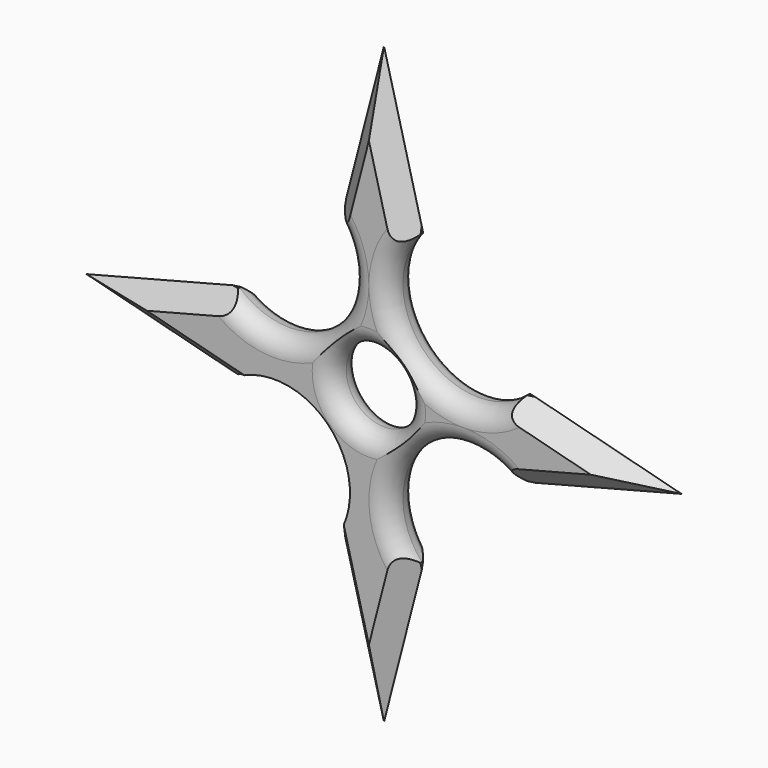
from build123d import *

# Parameters (mm, degrees)
F0_W         = 19.05
F0_H         = 25.4
F0_W_2       = 25.4
F0_H_2       = 19.05
F1_DEPTH     = 12.7
F3_D         = 50.8
F4_SIZE2     = 6.34999
F4_SIZE      = 6.34999
F5_T6_ANGLE  = 208.6059171241
F5_T8_ANGLE  = 208.6059171241
F5_T10_ANGLE = 208.6059171241
F5_T12_ANGLE = 208.6059171241
F5_T14_ANGLE = 208.6059171241
F5_T16_ANGLE = 208.6059171241
F5_T18_ANGLE = 208.6059171241


# Not quite as in the source:
# - a fillet or chamfer that OpenCascade refuses, or shapes differently, is made with other operations: its cross-section is extruded or revolved along the edge and cut away or added
# - a fillet or chamfer is up to 0.001 mm smaller than in the source, because OpenCascade refuses the exact size


with BuildPart() as f1:
    # F0 (on Front) → F1 (new body)
    with BuildSketch(Plane.XZ):
        with BuildLine():
            Line((-12.7, 12.7), (-4.87e-08, 12.7))
            Line((-4.87e-08, 12.7), (12.7, 12.7))
            Line((12.7, 12.7), (12.7, 14.1990316571))
            ThreePointArc((12.7, 14.1990316571), (0, 19.05), (-12.7, 14.1990316571))
            Line((-12.7, 14.1990316571), (-12.7, 12.7))
        make_face()
        with BuildLine():
            Line((-12.7, -12.7), (-12.7, 0))
            Line((-12.7, 0), (-12.7, 12.7))
            Line((-12.7, 12.7), (-14.1990316571, 12.7))
            ThreePointArc((-14.1990316571, 12.7), (-19.05, 0), (-14.1990316571, -12.7))
            Line((-14.1990316571, -12.7), (-12.7, -12.7))
        make_face()
        with BuildLine():
            Line((12.7, -12.7), (6e-10, -12.7))
            Line((6e-10, -12.7), (-12.7, -12.7))
            Line((-12.7, -12.7), (-12.7, -14.1990316571))
            ThreePointArc((-12.7, -14.1990316571), (0, -19.05), (12.7, -14.1990316571))
            Line((12.7, -14.1990316571), (12.7, -12.7))
        make_face()
        with BuildLine():
            Line((12.7, 12.7), (12.7, 0))
            Line((12.7, 0), (12.7, -12.7))
            Line((12.7, -12.7), (14.1990316571, -12.7))
            ThreePointArc((14.1990316571, -12.7), (17.7959834382, -6.7974608102), (19.05, 0))
            ThreePointArc((19.05, 0), (17.7959834382, 6.7974608102), (14.1990316571, 12.7))
            Line((14.1990316571, 12.7), (12.7, 12.7))
        make_face()
        with BuildLine():
            Line((12.7, -12.7), (12.7, 0))
            ThreePointArc((12.7, 0), (8.9802561213, -8.9802561208), (6e-10, -12.7))
            Line((6e-10, -12.7), (12.7, -12.7))
        make_face()
        with BuildLine():
            Line((-12.7, -12.7), (6e-10, -12.7))
            ThreePointArc((6e-10, -12.7), (-8.9802561208, -8.9802561213), (-12.7, 0))
            Line((-12.7, 0), (-12.7, -12.7))
        make_face()
        with BuildLine():
            ThreePointArc((-12.7, 0), (-8.9802561383, 8.9802561039), (-4.87e-08, 12.7))
            Line((-4.87e-08, 12.7), (-12.7, 12.7))
            Line((-12.7, 12.7), (-12.7, 0))
        make_face()
        with BuildLine():
            ThreePointArc((-4.87e-08, 12.7), (8.9802561039, 8.9802561383), (12.7, 0))
            Line((12.7, 0), (12.7, 12.7))
            Line((12.7, 12.7), (-4.87e-08, 12.7))
        make_face()
        with BuildLine():
            Line((12.7, 31.75), (12.7, 14.1990316571))
            ThreePointArc((12.7, 14.1990316571), (13.4703841816, 13.4703841816), (14.1990316571, 12.7))
            Line((14.1990316571, 12.7), (31.75, 12.7))
            Line((31.75, 12.7), (31.75, 31.75))
            Line((31.75, 31.75), (12.7, 31.75))
        make_face()
        with BuildLine():
            ThreePointArc((-12.7, 14.1990316571), (0, 19.05), (12.7, 14.1990316571))
            Line((12.7, 14.1990316571), (12.7, 31.75))
            Line((12.7, 31.75), (-12.7, 31.75))
            Line((-12.7, 31.75), (-12.7, 14.1990316571))
        make_face()
        with BuildLine():
            ThreePointArc((-14.1990316571, 12.7), (-13.4703841816, 13.4703841816), (-12.7, 14.1990316571))
            Line((-12.7, 14.1990316571), (-12.7, 31.75))
            Line((-12.7, 31.75), (-31.75, 31.75))
            Line((-31.75, 31.75), (-31.75, 12.7))
            Line((-31.75, 12.7), (-14.1990316571, 12.7))
        make_face()
        with BuildLine():
            ThreePointArc((-14.1990316571, -12.7), (-19.05, 0), (-14.1990316571, 12.7))
            Line((-14.1990316571, 12.7), (-31.75, 12.7))
            Line((-31.75, 12.7), (-31.75, -12.7))
            Line((-31.75, -12.7), (-14.1990316571, -12.7))
        make_face()
        with BuildLine():
            Line((-12.7, -31.75), (-12.7, -14.1990316571))
            ThreePointArc((-12.7, -14.1990316571), (-13.4703841816, -13.4703841816), (-14.1990316571, -12.7))
            Line((-14.1990316571, -12.7), (-31.75, -12.7))
            Line((-31.75, -12.7), (-31.75, -31.75))
            Line((-31.75, -31.75), (-12.7, -31.75))
        make_face()
        with BuildLine():
            Line((12.7, -31.75), (12.7, -14.1990316571))
            ThreePointArc((12.7, -14.1990316571), (0, -19.05), (-12.7, -14.1990316571))
            Line((-12.7, -14.1990316571), (-12.7, -31.75))
            Line((-12.7, -31.75), (12.7, -31.75))
        make_face()
        with BuildLine():
            ThreePointArc((14.1990316571, -12.7), (13.4703841816, -13.4703841816), (12.7, -14.1990316571))
            Line((12.7, -14.1990316571), (12.7, -31.75))
            Line((12.7, -31.75), (31.75, -31.75))
            Line((31.75, -31.75), (31.75, -12.7))
            Line((31.75, -12.7), (14.1990316571, -12.7))
        make_face()
        with BuildLine():
            ThreePointArc((19.05, 0), (17.7959834382, -6.7974608102), (14.1990316571, -12.7))
            Line((14.1990316571, -12.7), (31.75, -12.7))
            Line((31.75, -12.7), (31.75, 12.7))
            Line((31.75, 12.7), (14.1990316571, 12.7))
            ThreePointArc((14.1990316571, 12.7), (17.7959834382, 6.7974608102), (19.05, 0))
        make_face()
        with Locations((41.275, 0)):
            Rectangle(F0_W, F0_H)
        Polygon((50.8, 12.7), (50.8, -12.7), (99.9868884968, 0), align=None)
        Polygon((-12.7, 50.8), (12.7, 50.8), (0, 99.9868884968), align=None)
        with Locations((0, 41.275)):
            Rectangle(F0_W_2, F0_H_2)
        with Locations((-41.275, 0)):
            Rectangle(F0_W, F0_H)
        Polygon((-50.8, -12.7), (-50.8, 12.7), (-99.9868884968, 0), align=None)
        Polygon((0, -99.9868884968), (12.7, -50.8), (-12.7, -50.8), align=None)
        with Locations((0, -41.275)):
            Rectangle(F0_W_2, F0_H_2)
        with BuildLine():
            Line((14.1990316571, -12.7), (12.7, -12.7))
            Line((12.7, -12.7), (12.7, -14.1990316571))
            ThreePointArc((12.7, -14.1990316571), (13.4703841816, -13.4703841816), (14.1990316571, -12.7))
        make_face()
        with BuildLine():
            Line((-12.7, -14.1990316571), (-12.7, -12.7))
            Line((-12.7, -12.7), (-14.1990316571, -12.7))
            ThreePointArc((-14.1990316571, -12.7), (-13.4703841816, -13.4703841816), (-12.7, -14.1990316571))
        make_face()
        with BuildLine():
            Line((-14.1990316571, 12.7), (-12.7, 12.7))
            Line((-12.7, 12.7), (-12.7, 14.1990316571))
            ThreePointArc((-12.7, 14.1990316571), (-13.4703841816, 13.4703841816), (-14.1990316571, 12.7))
        make_face()
        with BuildLine():
            Line((12.7, 14.1990316571), (12.7, 12.7))
            Line((12.7, 12.7), (14.1990316571, 12.7))
            ThreePointArc((14.1990316571, 12.7), (13.4703841816, 13.4703841816), (12.7, 14.1990316571))
        make_face()
    extrude(amount=F1_DEPTH)

    # F3 (through all)
    with Locations(Plane.XZ.offset(12.7)):
        with Locations((-31.75, 31.75), (-31.75, -31.75), (31.75, -31.75), (31.75, 31.75)):
            Hole(F3_D / 2)

    # F4 (size 6.35 and 6.35 in the source; OpenCascade refuses exactly that, so slightly less here)
    f4_edges = [f1.edges().sort_by_distance(p)[0] for p in [
        (-75.393444, -12.7, 6.35),
        (-75.393444, -12.7, -6.35),
        (-75.393444, 0, -6.35),
        (-75.393444, 0, 6.35),
        (6.35, -12.7, 75.393444),
        (-6.35, -12.7, 75.393444),
        (-6.35, 0, 75.393444),
        (6.35, 0, 75.393444),
        (75.393444, 0, 6.35),
        (75.393444, -12.7, 6.35),
        (75.393444, 0, -6.35),
        (75.393444, -12.7, -6.35),
        (-6.35, 0, -75.393444),
        (6.35, 0, -75.393444),
        (6.35, -12.7, -75.393444),
        (-6.35, -12.7, -75.393444),
    ]]
    chamfer(f4_edges, length=F4_SIZE, length2=F4_SIZE2)

    # F5: fillet of radius 6.35 on 9 edges, made by hand

    # F5_s1 → F5_t2 (revolve, cut)
    with BuildSketch(Plane.YZ):
        with BuildLine():
            ThreePointArc((-6.35, 12.7), (-1.8598719395, 14.5598719395), (0, 19.05))
            Line((0, 19.05), (0, 12.7))
            Line((0, 12.7), (-6.35, 12.7))
        make_face()
    revolve(axis=Axis((0, 0, 0), (0, 1, 0)), mode=Mode.SUBTRACT)

    # F5_s3 → F5_t4 (revolve, cut)
    with BuildSketch(Plane.YZ):
        with BuildLine():
            ThreePointArc((-12.7, 19.05), (-10.8401280605, 14.5598719395), (-6.35, 12.7))
            Line((-6.35, 12.7), (-12.7, 12.7))
            Line((-12.7, 12.7), (-12.7, 19.05))
        make_face()
    revolve(axis=Axis((0, -12.7, 0), (0, 1, 0)), mode=Mode.SUBTRACT)

    # F5_s5 → F5_t6 (revolve, cut)
    with BuildSketch(Plane(origin=(-37.4128674881, 0, 22.2115222373), x_dir=(0, 1, 0), z_dir=(-0.8598786332, 0, 0.5104985173))):
        with BuildLine():
            ThreePointArc((-12.7, -42.8428186777), (-10.8401280605, -38.3526906172), (-6.35, -36.4928186777))
            Line((-6.35, -36.4928186777), (-12.7, -36.4928186777))
            Line((-12.7, -36.4928186777), (-12.7, -42.8428186777))
        make_face()
    revolve(axis=Axis((-31.75, -12.7, 31.75), (0, 1, 0)), revolution_arc=F5_T6_ANGLE, mode=Mode.SUBTRACT)

    # F5_s7 → F5_t8 (revolve, cut)
    with BuildSketch(Plane(origin=(37.4128674881, 0, 22.2115222373), x_dir=(0, 1, 0), z_dir=(0.8598786332, 0, 0.5104985173))):
        with BuildLine():
            ThreePointArc((-12.7, 42.8428186777), (-10.8401280605, 38.3526906172), (-6.35, 36.4928186777))
            Line((-6.35, 36.4928186777), (-12.7, 36.4928186777))
            Line((-12.7, 36.4928186777), (-12.7, 42.8428186777))
        make_face()
    revolve(axis=Axis((31.75, -12.7, 31.75), (0, -1, 0)), revolution_arc=F5_T8_ANGLE, mode=Mode.SUBTRACT)

    # F5_s9 → F5_t10 (revolve, cut)
    with BuildSketch(Plane(origin=(22.2115222373, 0, -37.4128674881), x_dir=(0, 1, 0), z_dir=(0.5104985173, 0, -0.8598786332))):
        with BuildLine():
            ThreePointArc((-12.7, 42.8428186777), (-10.8401280605, 38.3526906172), (-6.35, 36.4928186777))
            Line((-6.35, 36.4928186777), (-12.7, 36.4928186777))
            Line((-12.7, 36.4928186777), (-12.7, 42.8428186777))
        make_face()
    revolve(axis=Axis((31.75, -12.7, -31.75), (0, -1, 0)), revolution_arc=F5_T10_ANGLE, mode=Mode.SUBTRACT)

    # F5_s11 → F5_t12 (revolve, cut)
    with BuildSketch(Plane(origin=(-22.2115222373, 0, 37.4128674881), x_dir=(0, 1, 0), z_dir=(-0.5104985173, 0, 0.8598786332))):
        with BuildLine():
            ThreePointArc((-6.35, 36.4928186777), (-1.8598719395, 38.3526906172), (0, 42.8428186777))
            Line((0, 42.8428186777), (0, 36.4928186777))
            Line((0, 36.4928186777), (-6.35, 36.4928186777))
        make_face()
    revolve(axis=Axis((-31.75, 0, 31.75), (0, -1, 0)), revolution_arc=F5_T12_ANGLE, mode=Mode.SUBTRACT)

    # F5_s13 → F5_t14 (revolve, cut)
    with BuildSketch(Plane(origin=(37.4128674881, 0, 22.2115222373), x_dir=(0, 1, 0), z_dir=(0.8598786332, 0, 0.5104985173))):
        with BuildLine():
            ThreePointArc((-6.35, 36.4928186777), (-1.8598719395, 38.3526906172), (0, 42.8428186777))
            Line((0, 42.8428186777), (0, 36.4928186777))
            Line((0, 36.4928186777), (-6.35, 36.4928186777))
        make_face()
    revolve(axis=Axis((31.75, 0, 31.75), (0, -1, 0)), revolution_arc=F5_T14_ANGLE, mode=Mode.SUBTRACT)

    # F5_s15 → F5_t16 (revolve, cut)
    with BuildSketch(Plane(origin=(-37.4128674881, 0, -22.2115222373), x_dir=(0, 1, 0), z_dir=(-0.8598786332, 0, -0.5104985173))):
        with BuildLine():
            ThreePointArc((-6.35, 36.4928186777), (-1.8598719395, 38.3526906172), (0, 42.8428186777))
            Line((0, 42.8428186777), (0, 36.4928186777))
            Line((0, 36.4928186777), (-6.35, 36.4928186777))
        make_face()
    revolve(axis=Axis((-31.75, 0, -31.75), (0, -1, 0)), revolution_arc=F5_T16_ANGLE, mode=Mode.SUBTRACT)

    # F5_s17 → F5_t18 (revolve, cut)
    with BuildSketch(Plane(origin=(22.2115222373, 0, -37.4128674881), x_dir=(0, 1, 0), z_dir=(0.5104985173, 0, -0.8598786332))):
        with BuildLine():
            ThreePointArc((-6.35, 36.4928186777), (-1.8598719395, 38.3526906172), (0, 42.8428186777))
            Line((0, 42.8428186777), (0, 36.4928186777))
            Line((0, 36.4928186777), (-6.35, 36.4928186777))
        make_face()
    revolve(axis=Axis((31.75, 0, -31.75), (0, -1, 0)), revolution_arc=F5_T18_ANGLE, mode=Mode.SUBTRACT)


solid = f1.part
